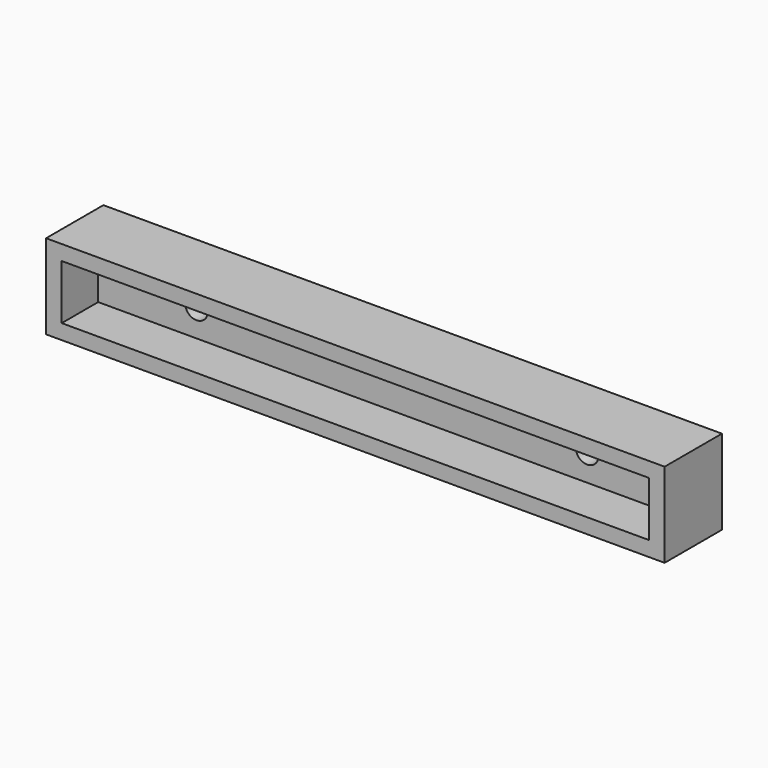
from build123d import *

# Parameters (mm, degrees)
F0_W     = 95
F0_H     = 13
F1_DEPTH = 11
F2_W     = 90.2
F2_H     = 8.4
F3_DEPTH = 7
F4_R     = 1.75
F5_DEPTH = 4


# Not quite as in the source:
# - a pattern or mirror of a feature is missing from the dataset's text; its kind, count and spacing are read off the source's solid


with BuildPart() as f1:
    # F0 (on Front) → F1 (new body)
    with BuildSketch(Plane.XZ):
        Rectangle(F0_W, F0_H)
    extrude(amount=F1_DEPTH)

    # F2 (on face) → F3 (cut)
    with BuildSketch(Plane.XZ.offset(11)):
        Rectangle(F2_W, F2_H)
    extrude(amount=-F3_DEPTH, mode=Mode.SUBTRACT)

    # F4 (on face) → F5 (cut, through all)
    with BuildSketch(Plane.XZ.offset(4)):
        with Locations((-30, 0)):
            Circle(F4_R)
    f5 = extrude(amount=-F5_DEPTH, mode=Mode.SUBTRACT)

    # F5_copies: F5 across plane
    add(f5.mirror(Plane(origin=(0, 0, 0), x_dir=(0, 0, 1), z_dir=(1, 0, 0))), mode=Mode.SUBTRACT)


solid = f1.part
